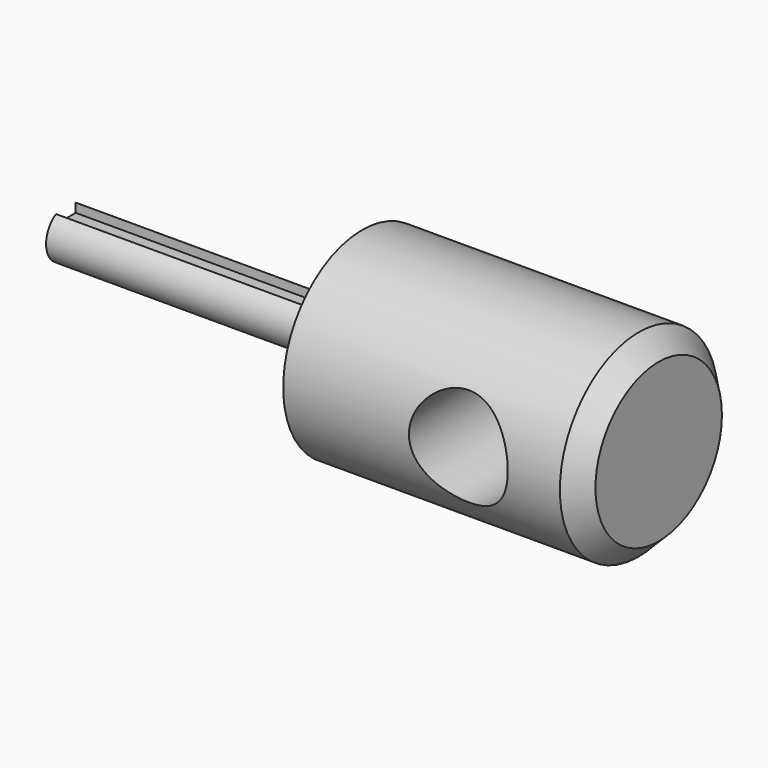
from build123d import *

# Parameters (mm, degrees)
F1_DEPTH = 76.2
F2_R     = 25.4
F3_DEPTH = 76.2
F4_R     = 2.65
F5_DEPTH = 25.4
F6_R     = 12.7
F7_DEPTH = 25.4
F8_SIZE  = 5.08


with BuildPart() as f1:
    # F0 (on Right) → F1 (new body)
    with BuildSketch(Plane.YZ):
        with BuildLine():
            Line((-3.175, 3.175), (-3.175, 5.499261314))
            ThreePointArc((-3.175, 5.499261314), (0, -6.35), (3.175, 5.499261314))
            Line((3.175, 5.499261314), (3.175, 3.175))
            Line((3.175, 3.175), (-3.175, 3.175))
        make_face()
    extrude(amount=F1_DEPTH)

    # F2 (on face) → F3 (join)
    with BuildSketch(Plane.YZ.offset(76.2)):
        Circle(F2_R)
    extrude(amount=F3_DEPTH)

    # F4 (on face) → F5 (cut)
    with BuildSketch(Plane(origin=(0, 0, 0), x_dir=(0, -1, 0), z_dir=(-1, 0, 0))):
        Circle(F4_R)
    extrude(amount=-F5_DEPTH, mode=Mode.SUBTRACT)

    # F6 (on Front) → F7 (cut, symmetric)
    with BuildSketch(Plane.XZ):
        with Locations((121.220822216, 0)):
            Circle(F6_R)
    extrude(amount=F7_DEPTH, both=True, mode=Mode.SUBTRACT)

    # F8
    f8_edges = [f1.edges().sort_by_distance(p)[0] for p in [
        (152.4, -25.4, 0),
    ]]
    chamfer(f8_edges, length=F8_SIZE)


solid = f1.part
